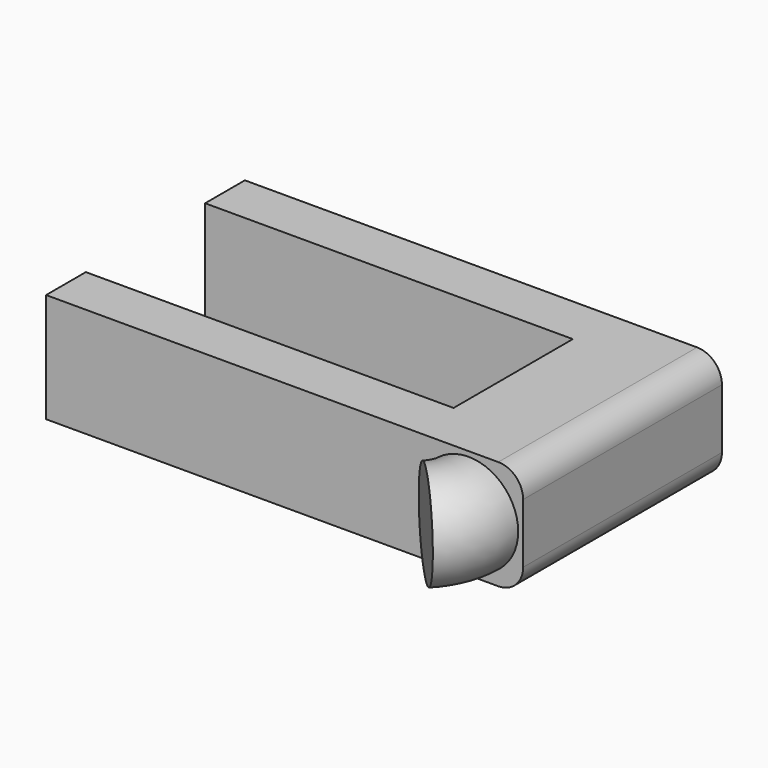
from build123d import *

# Parameters (mm, degrees)
F0_R     = 10
F2_ANGLE = 45
F3_W     = 22
F3_H     = 22
F3_R     = 10
F4_DEPTH = 50
F5_W     = 10
F5_H     = 22
F6_DEPTH = 74
F7_W     = 10
F7_H     = 22
F8_DEPTH = 74
F9_R     = 5


with BuildPart() as f2:
    # F0 (on Front) → F2 (revolve)
    with BuildSketch(Plane.XZ):
        Circle(F0_R)
    revolve(axis=Axis((-10.0093111396, 0, -0.720274169), (0, 0, -1)), revolution_arc=F2_ANGLE)

    # F3 (on face) → F4 (join)
    with BuildSketch(Plane(origin=(0, 0, 0), x_dir=(-1, 0, 0), z_dir=(0, 1, 0))):
        Rectangle(F3_W, F3_H)
        Circle(F3_R, mode=Mode.SUBTRACT)
        Circle(F3_R)
    extrude(amount=F4_DEPTH)

    # F5 (on face) → F6 (join)
    with BuildSketch(Plane(origin=(-11, 0, 0), x_dir=(0, -1, 0), z_dir=(-1, 0, 0))):
        with Locations((-5, 0)):
            Rectangle(F5_W, F5_H)
    extrude(amount=F6_DEPTH)

    # F7 (on face) → F8 (join)
    with BuildSketch(Plane(origin=(-11, 0, 0), x_dir=(0, -1, 0), z_dir=(-1, 0, 0))):
        with Locations((-45, 0)):
            Rectangle(F7_W, F7_H)
    extrude(amount=F8_DEPTH)

    # F9
    f9_edges = [f2.edges().sort_by_distance(p)[0] for p in [
        (11, 25, -11),
        (11, 25, 11),
    ]]
    fillet(f9_edges, radius=F9_R)


solid = f2.part
